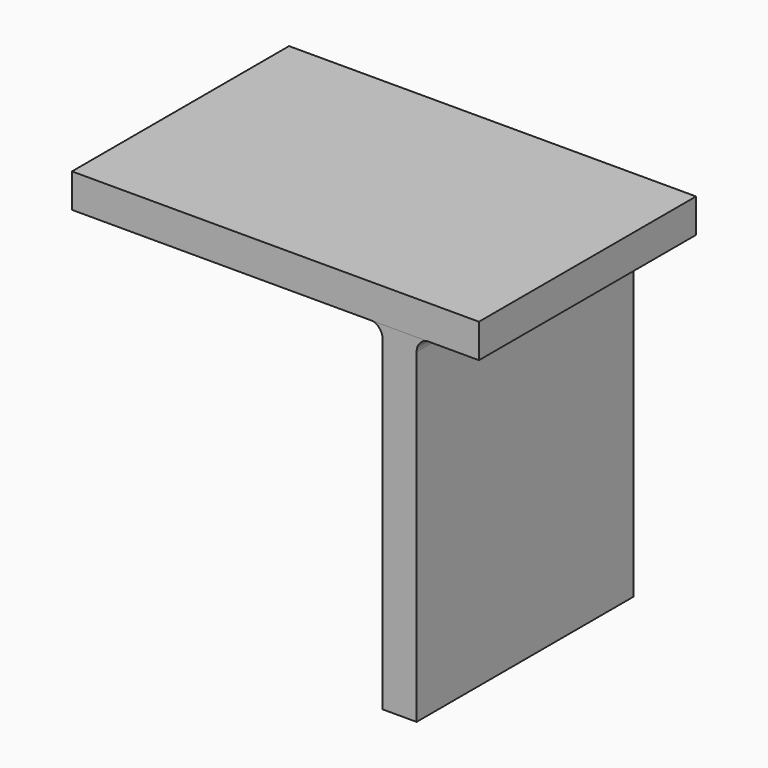
from build123d import *

# Parameters (mm, degrees)
F0_W     = 76.2
F0_H     = 50.8
F1_DEPTH = 6.35
F3_W     = 50.8
F3_H     = 63.5
F4_DEPTH = 6.35
F5_R     = 2.5


with BuildPart() as f1:
    # F0 (on Top) → F1 (new body)
    with BuildSketch(Plane.XY):
        with Locations((1.0298034176, -8.9605891951)):
            Rectangle(F0_W, F0_H)
    extrude(amount=F1_DEPTH)

    # F3 (on offset) → F4 (join)
    with BuildSketch(Plane.YZ.offset(21)):
        with Locations((-8.8295020819, -31.75)):
            Rectangle(F3_W, F3_H)
    extrude(amount=F4_DEPTH)

    # F5
    f5_edges = [f1.edges().sort_by_distance(p)[0] for p in [
        (21, -8.895046, 0),
        (27.35, -8.895046, 0),
    ]]
    fillet(f5_edges, radius=F5_R)


solid = f1.part
